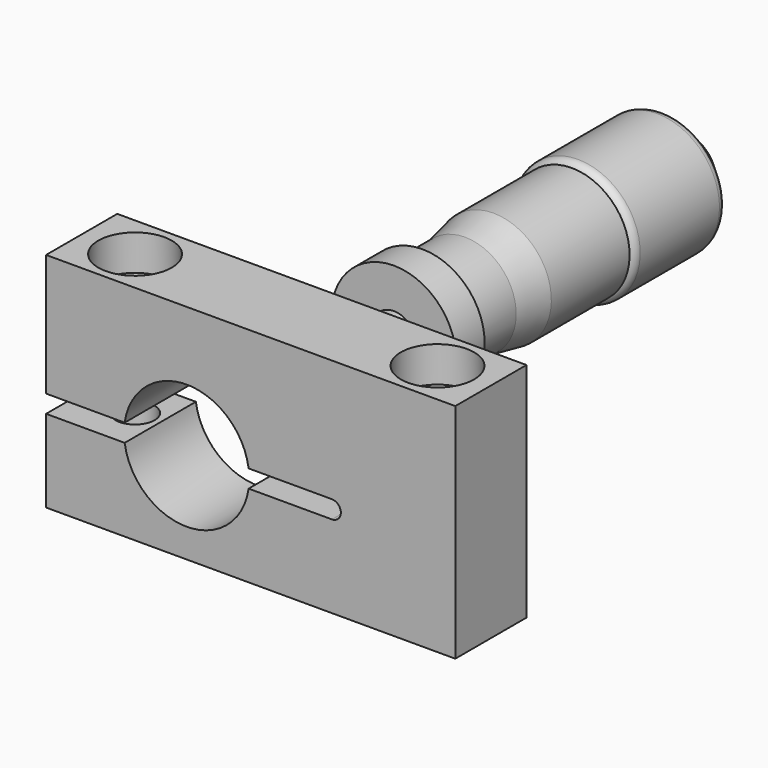
from build123d import *

# Parameters (mm, degrees)
F3_R           = 2.5
F6_DEPTH       = 10
F8_D           = 4.4
F8_CBORE_D     = 8.25
F8_CBORE_DEPTH = 4


# Not quite as in the source:
# - a fillet or chamfer that OpenCascade refuses, or shapes differently, is made with other operations: its cross-section is extruded or revolved along the edge and cut away or added


with BuildPart() as f1:
    # F0 (on Right) → F1 (revolve)
    with BuildSketch(Plane.YZ):
        Polygon((8.0745064616, 6.5), (4.0745064616, 5.75), (-1.9254935384, 5.75), (-1.9254935384, 7), (-5.9254935384, 7), (-5.9254935384, 2.5), (-16.9254935384, 2.5), (-16.9254935384, 0), (35.0745064616, 0), (35.0745064616, 4), (32.0745064616, 4), (32.0745064616, 7), (19.0745064616, 7), (19.0745064616, 6.5), align=None)
    revolve(axis=Axis((0, 9.0745064616, 0), (0, 1, 0)))

    # F2: fillet of radius 1 on 3 edges, made by hand

    # F2_s1 → F2_t2 (revolve, cut)
    with BuildSketch(Plane.YZ):
        with BuildLine():
            ThreePointArc((35.0745064616, 3), (34.7816132428, 3.7071067812), (34.0745064616, 4))
            Line((34.0745064616, 4), (34.0745064616, 4.02))
            Line((34.0745064616, 4.02), (35.0945064616, 4.02))
            Line((35.0945064616, 4.02), (35.0945064616, 3))
            Line((35.0945064616, 3), (35.0745064616, 3))
        make_face()
    revolve(axis=Axis((0, 35.0745064616, 0), (0, 1, 0)), mode=Mode.SUBTRACT)

    # F2_s3 → F2_t4 (revolve, cut)
    with BuildSketch(Plane.YZ):
        with BuildLine():
            ThreePointArc((32.0745064616, 6), (31.7816132428, 6.7071067812), (31.0745064616, 7))
            Line((31.0745064616, 7), (31.0745064616, 7.02))
            Line((31.0745064616, 7.02), (32.0945064616, 7.02))
            Line((32.0945064616, 7.02), (32.0945064616, 6))
            Line((32.0945064616, 6), (32.0745064616, 6))
        make_face()
    revolve(axis=Axis((0, 32.0745064616, 0), (0, 1, 0)), mode=Mode.SUBTRACT)

    # F2_s5 → F2_t6 (revolve, cut)
    with BuildSketch(Plane.YZ):
        with BuildLine():
            ThreePointArc((19.9405318654, 7), (19.4405318654, 6.8660254038), (19.0745064616, 6.5))
            Line((19.0745064616, 6.5), (19.0571859535, 6.51))
            ThreePointArc((19.0571859535, 6.51), (19.0545064616, 6.75), (19.0545064616, 7))
            Line((19.0545064616, 7), (19.0745064616, 7.02))
            Line((19.0745064616, 7.02), (19.9405318654, 7.02))
            Line((19.9405318654, 7.02), (19.9405318654, 7))
        make_face()
    revolve(axis=Axis((0, 19.0745064616, 0), (0, 1, 0)), mode=Mode.SUBTRACT)

    # F3
    f3_edges = [f1.edges().sort_by_distance(p)[0] for p in [
        (0, -16.925494, -2.5),
    ]]
    fillet(f3_edges, radius=F3_R)


with BuildPart() as f6:
    # F5 (on offset) → F6 (new body)
    with BuildSketch(Plane.XZ.offset(25)):
        with BuildLine():
            Line((-15.8362010978, -10.2766921259), (30.1637989022, -10.2766921259))
            Line((30.1637989022, -10.2766921259), (30.1637989022, 14.7233078741))
            Line((30.1637989022, 14.7233078741), (-15.8362010978, 14.7233078741))
            Line((-15.8362010978, 14.7233078741), (-15.8362010978, 1))
            Line((-15.8362010978, 1), (-7.0018163238, 1))
            ThreePointArc((-7.0018163238, 1), (-0.0350231516, 7.0381962962), (6.9317700206, 1))
            Line((6.9317700206, 1), (16.2971732207, 1))
            ThreePointArc((16.2971732207, 1), (17.2971732207, 0), (16.2971732207, -1))
            Line((16.2971732207, -1), (6.9317700206, -1))
            ThreePointArc((6.9317700206, -1), (-0.0350231516, -7.0381962962), (-7.0018163238, -1))
            Line((-7.0018163238, -1), (-15.8362010978, -1))
            Line((-15.8362010978, -1), (-15.8362010978, -10.2766921259))
        make_face()
    extrude(amount=F6_DEPTH)

    # F8 (through all)
    with Locations(Plane.XY.offset(14.7233078741)):
        with Locations((24.1637989022, -30), (-9.8362010978, -30)):
            CounterBoreHole(F8_D / 2, F8_CBORE_D / 2, F8_CBORE_DEPTH)


solid = Compound([f1.part, f6.part])
